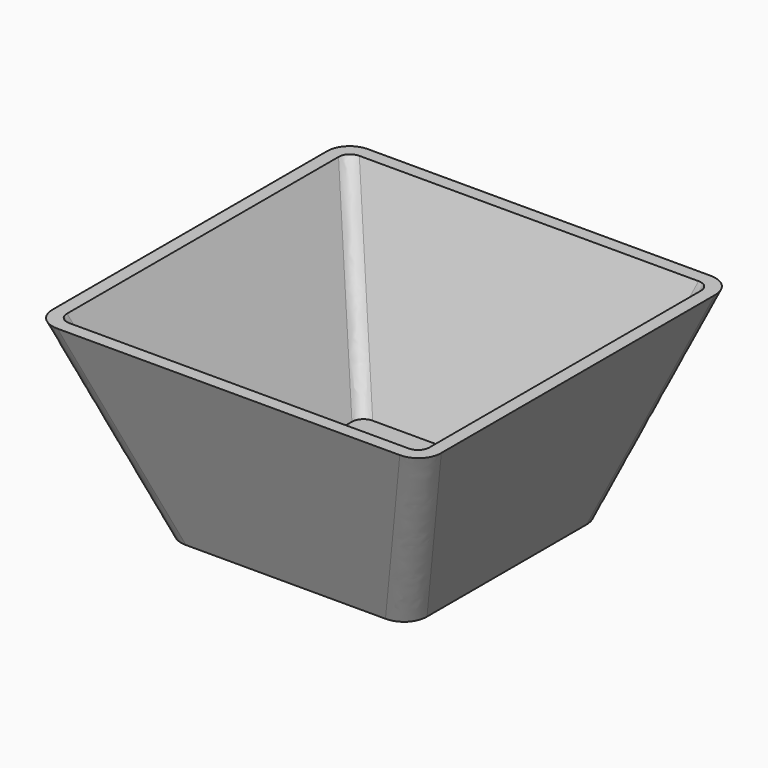
from build123d import *

# Parameters (mm, degrees)
F0_W     = 50
F0_H     = 50
F1_DEPTH = 40
F1_TAPER = -20
F2_R     = 5
F3_T     = -2.5
F4_R     = 20
F5_DEPTH = 1.5


with BuildPart() as f1:
    # F0 (on Top) → F1 (new body)
    with BuildSketch(Plane.XY):
        Rectangle(F0_W, F0_H)
    extrude(amount=F1_DEPTH, taper=F1_TAPER)

    # F2
    f2_edges = [f1.edges().sort_by_distance(p)[0] for p in [
        (32.279405, 32.279405, 20),
        (-32.279405, 32.279405, 20),
        (32.279405, -32.279405, 20),
        (-32.279405, -32.279405, 20),
    ]]
    fillet(f2_edges, radius=F2_R)

    # F3
    f3_openings = [f1.faces().sort_by_distance(p)[0] for p in [
        (0, 0, 40),
    ]]
    offset(amount=F3_T, openings=f3_openings)

    # F4 (on face) → F5 (cut)
    with BuildSketch(Plane.XY.offset(2.5)):
        Circle(F4_R)
    extrude(amount=-F5_DEPTH, mode=Mode.SUBTRACT)


solid = f1.part
